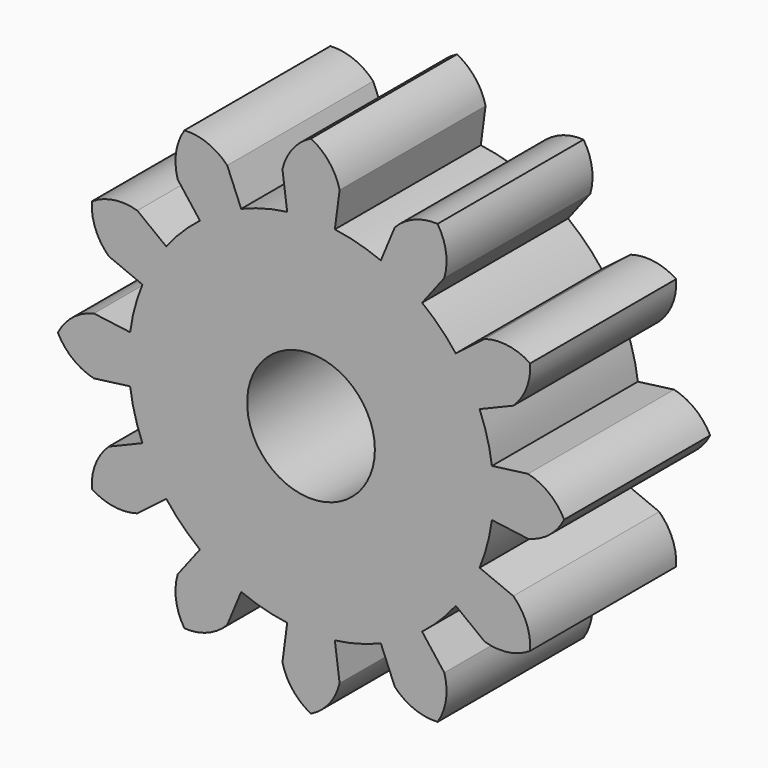
from build123d import *

# Parameters (mm, degrees)
F2_DEPTH        = 10
F2_COPIES_COUNT = 12
F4_R            = 7
F5_DEPTH        = 20.001


# Not quite as in the source:
# - a feature of the source that left no trace in its solid (it failed there, or was rolled back) is left out
# - a pattern or mirror of a feature is missing from the dataset's text; its kind, count and spacing are read off the source's solid


with BuildPart() as f2:
    # F1 (on Front) → F2 (new body, symmetric)
    with BuildSketch(Plane.XZ):
        with BuildLine():
            ThreePointArc((-2.6105238444, 19.8288972275), (-13.186916302, -15.0367961496), (20, 0))
            ThreePointArc((20, 0), (15.0367961496, 13.186916302), (2.6105238444, 19.8288972275))
            ThreePointArc((2.6105238444, 19.8288972275), (0, 20), (-2.6105238444, 19.8288972275))
        make_face()
        with BuildLine():
            ThreePointArc((-2.6105238444, 19.8288972275), (0, 20), (2.6105238444, 19.8288972275))
            Line((2.6105238444, 19.8288972275), (3.1326286133, 23.794676673))
            ThreePointArc((3.1326286133, 23.794676673), (2.0019466325, 26.1165955987), (0, 27.7481466766))
            ThreePointArc((0, 27.7481466766), (-2.0019466325, 26.1165955987), (-3.1326286133, 23.794676673))
            Line((-3.1326286133, 23.794676673), (-2.6105238444, 19.8288972275))
        make_face()
    extrude(amount=F2_DEPTH, both=True)

    # F2_copies: F2 ×12 about axis
    f2_copies_axis = Axis((0, 0, 0), (0, 1, 0))


with BuildPart() as f2_1:
    add(f2.part)
    for i in range(1, F2_COPIES_COUNT):
        add(f2.part.rotate(f2_copies_axis, i * 360 / F2_COPIES_COUNT))

    # F4 (on face) → F5 (cut, through all)
    with BuildSketch(Plane.XZ.offset(10)):
        Circle(F4_R)
    extrude(amount=-F5_DEPTH, mode=Mode.SUBTRACT)


solid = f2_1.part
